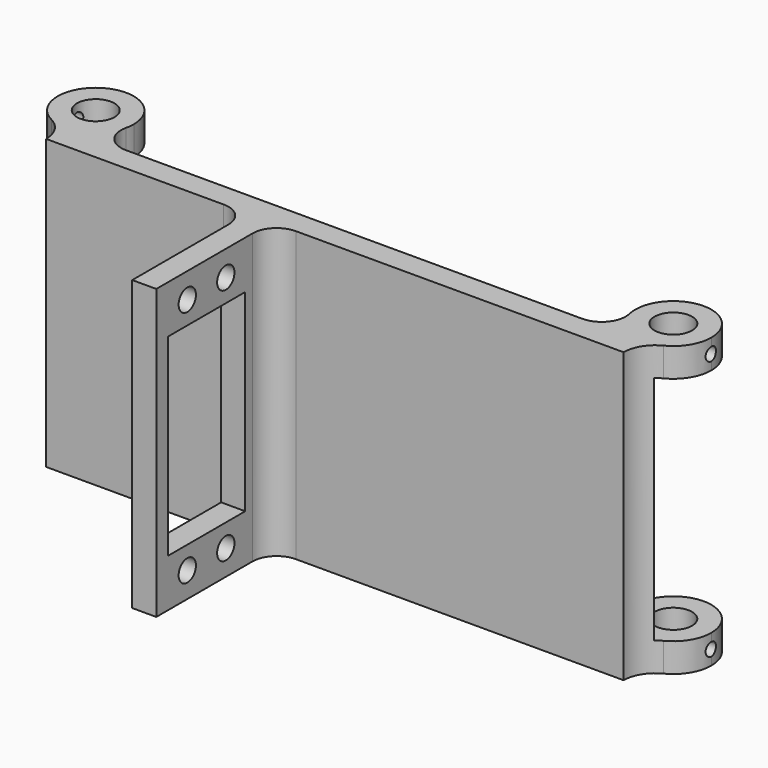
from build123d import *

# Parameters (mm, degrees)
F0_R          = 3.9
F0_W          = 5
F0_H          = 30
F1_DEPTH      = 60
F2_W          = 20.1
F2_H          = 40.1
F2_R          = 2.25
F3_DEPTH      = 54.801
F5_W          = 34.2169012874
F5_H          = 48
F6_DEPTH      = 67.901
F6_DEPTH_BACK = 67.901
F7_R          = 5
F9_R          = 1.35
F10_DEPTH     = 7.901


# Not quite as in the source:
# - a pattern or mirror of a feature is missing from the dataset's text; its kind, count and spacing are read off the source's solid


with BuildPart() as f1:
    # F0 (on Top) → F1 (new body)
    with BuildSketch(Plane.XY):
        with BuildLine():
            ThreePointArc((-52.3022123868, 6.1240310078), (-55.0816748297, 1.717761124), (-60, 0))
            Line((-60, 0), (-47.43019491, 0))
            ThreePointArc((-47.43019491, 0), (-51.3430043252, 1.8871359682), (-52.3022123868, 6.1240310078))
        make_face()
        Polygon((-47.43019491, 0), (-60, 0), (-60, -5), (-18.1, -5), (-13.1, -5), (60, -5), (60, 0), (47.43019491, 0), align=None)
        with BuildLine():
            Line((-60, -5), (-60, 0))
            ThreePointArc((-60, 0), (-61.846439606, 0.218811239), (-63.5905952277, 0.8631238528))
            ThreePointArc((-63.5905952277, 0.8631238528), (-60.9689691941, -1.5623919871), (-60, -5))
        make_face()
        with BuildLine():
            ThreePointArc((-63.5905952277, 0.8631238528), (-61.846439606, 0.218811239), (-60, 0))
            ThreePointArc((-60, 0), (-55.0816748297, 1.717761124), (-52.3022123868, 6.1240310078))
            ThreePointArc((-52.3022123868, 6.1240310078), (-52.1507158879, 7.0062780479), (-52.1, 7.9))
            ThreePointArc((-52.1, 7.9), (-64.125790694, 14.6370506269), (-63.5905952277, 0.8631238528))
        make_face()
        with Locations((-60, 7.9)):
            Circle(F0_R, mode=Mode.SUBTRACT)
        with BuildLine():
            ThreePointArc((52.3022123868, 6.1240310078), (51.3430043252, 1.8871359682), (47.43019491, 0))
            Line((47.43019491, 0), (60, 0))
            ThreePointArc((60, 0), (55.0816748297, 1.717761124), (52.3022123868, 6.1240310078))
        make_face()
        with Locations((-15.6, -20)):
            Rectangle(F0_W, F0_H)
        with BuildLine():
            ThreePointArc((63.5905952277, 0.8631238528), (61.846439606, 0.218811239), (60, 0))
            Line((60, 0), (60, -5))
            ThreePointArc((60, -5), (60.9689691941, -1.5623919871), (63.5905952277, 0.8631238528))
        make_face()
        with BuildLine():
            ThreePointArc((52.3022123868, 6.1240310078), (55.0816748297, 1.717761124), (60, 0))
            ThreePointArc((60, 0), (61.846439606, 0.218811239), (63.5905952277, 0.8631238528))
            ThreePointArc((63.5905952277, 0.8631238528), (66.7370506269, 3.774209306), (67.9, 7.9))
            ThreePointArc((67.9, 7.9), (59.1062780479, 15.7492841121), (52.3022123868, 6.1240310078))
        make_face()
        with Locations((60, 7.9)):
            Circle(F0_R, mode=Mode.SUBTRACT)
    extrude(amount=F1_DEPTH)

    # F2 (on face) → F3 (cut, through all)
    with BuildSketch(Plane.YZ.offset(-13.1)):
        with Locations((-21.95, 30)):
            Rectangle(F2_W, F2_H)
        with Locations((-26.95, 54.75)):
            Circle(F2_R)
        with Locations((-16.95, 54.75)):
            Circle(F2_R)
        with Locations((-16.95, 5.25)):
            Circle(F2_R)
        with Locations((-26.95, 5.25)):
            Circle(F2_R)
    extrude(amount=-F3_DEPTH, mode=Mode.SUBTRACT)

    # F5 (on Right) → F6 (cut, two sides)
    with BuildSketch(Plane.YZ) as f6_sk:
        with Locations((17.1084506437, 30)):
            Rectangle(F5_W, F5_H)
    extrude(amount=-F6_DEPTH, mode=Mode.SUBTRACT)
    extrude(f6_sk.sketch, amount=F6_DEPTH_BACK, mode=Mode.SUBTRACT)

    # F7
    f7_edges = [f1.edges().sort_by_distance(p)[0] for p in [
        (-13.1, -5, 30),
        (-18.1, -5, 30),
    ]]
    fillet(f7_edges, radius=F7_R)

    # F9 (on offset) → F10 (cut, through all)
    with BuildSketch(Plane.YZ.offset(60)):
        with Locations((7.9, 57)):
            Circle(F9_R)
        with Locations((7.9, 3)):
            Circle(F9_R)
    f10 = extrude(amount=F10_DEPTH, mode=Mode.SUBTRACT)

    # F10_copies: F10 across plane
    add(f10.mirror(Plane(origin=(-5e-06, 0, 0), x_dir=(0, 0, -1), z_dir=(-1, 0, 0))), mode=Mode.SUBTRACT)


solid = f1.part
